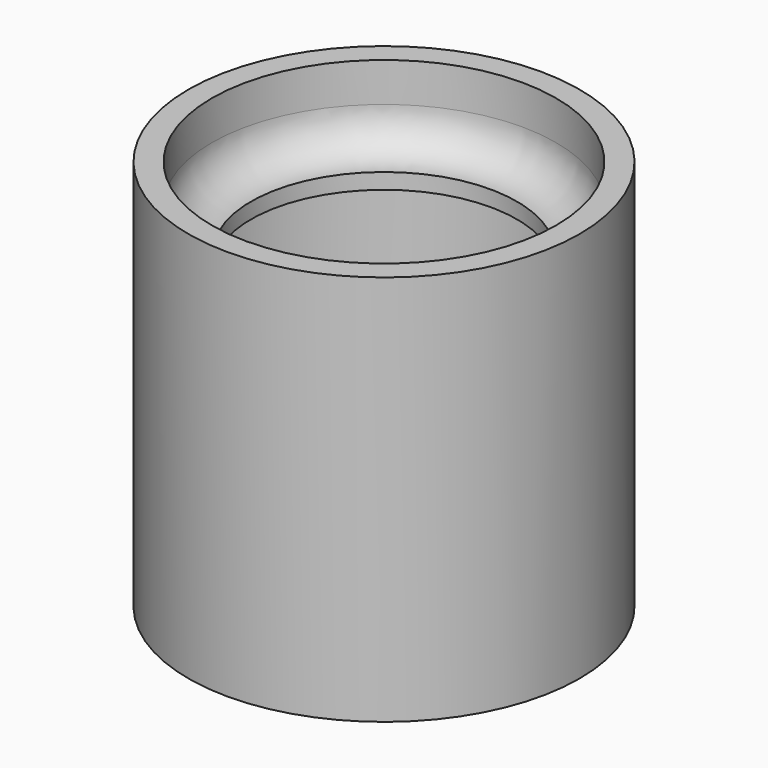
from build123d import *

# Parameters (mm, degrees)
F0_R     = 25
F1_DEPTH = 50
F2_R     = 22
F3_DEPTH = 10
F4_R     = 5
F5_T     = 2


# Not quite as in the source:
# - a shell that OpenCascade refuses in one call is made with other operations: the cavity is built on its own and cut out


with BuildPart() as f1:
    # F0 (on Top) → F1 (new body)
    with BuildSketch(Plane.XY):
        Circle(F0_R)
    extrude(amount=F1_DEPTH)

    # F2 (on face) → F3 (cut)
    with BuildSketch(Plane.XY.offset(50)):
        Circle(F2_R)
    extrude(amount=-F3_DEPTH, mode=Mode.SUBTRACT)

    # F4
    f4_edges = [f1.edges().sort_by_distance(p)[0] for p in [
        (-22, 0, 40),
    ]]
    fillet(f4_edges, radius=F4_R)

    # F5: shell of thickness 2, made by hand


with BuildPart() as f5_core1:
    # F5_t2: copy of F1
    add(f1.part)

    # the walls: a layer under each face that stays
    f5_faces = [f5_core1.faces().sort_by_distance(p)[0] for p in [
        (-22, 0, 47.5),
        (-20.5355339059, 0, 41.4644660941),
        (-16.6666666667, -16.6666666667, 50),
        (-25, 0, 25),
        (0, 0, 0),
    ]]
    thicken(f5_faces, amount=-F5_T, mode=Mode.SUBTRACT)


with BuildPart() as f1_1:
    add(f1.part)

    # what is left inside the walls is the cavity
    f5_cavity = [f5_core1.part.solids().sort_by_distance(p)[0] for p in [
        (-22.98, 0, 28.262966),
    ]]
    add(f5_cavity, mode=Mode.SUBTRACT)


solid = f1_1.part
